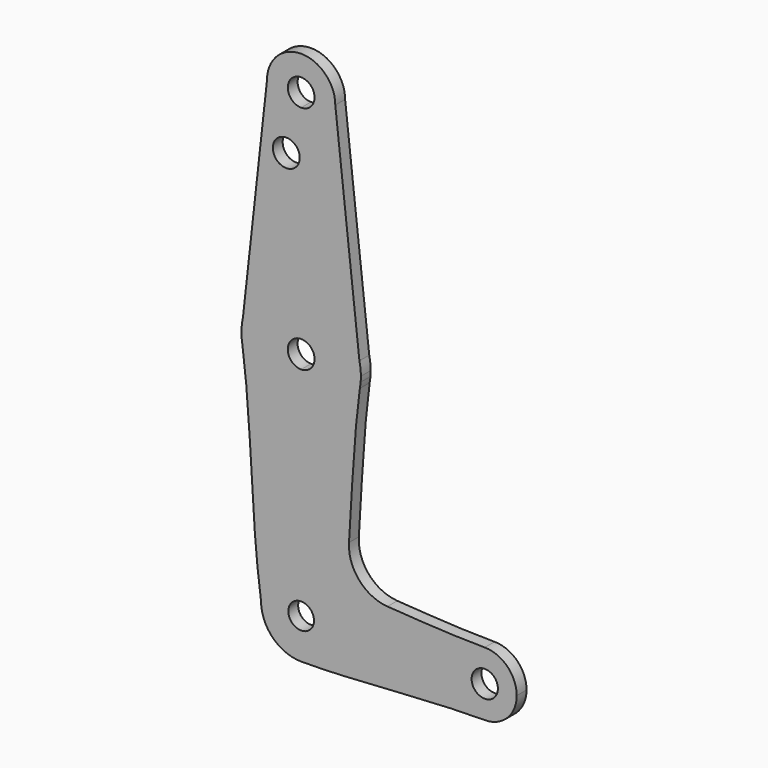
from build123d import *

# Parameters (mm, degrees)
F0_R     = 3.338805446
F1_DEPTH = 3.048


with BuildPart() as f1:
    # F0 (on Front) → F1 (new body)
    with BuildSketch(Plane.XZ):
        with BuildLine():
            ThreePointArc((-48.8398405267, 60.6527402997), (-46.3601680284, 54.6662813241), (-40.3737090528, 52.1866088258))
            ThreePointArc((-40.3737090528, 52.1866088258), (-34.3872500772, 54.6662813241), (-31.9075775789, 60.6527402997))
            ThreePointArc((-31.9075775789, 60.6527402997), (-40.3737090528, 69.1188717736), (-48.8398405267, 60.6527402997))
        make_face()
        with BuildLine():
            ThreePointArc((-37.0553247631, 60.6527402997), (-38.0272570189, 58.3062882658), (-40.3737090528, 57.33435601))
            ThreePointArc((-40.3737090528, 57.33435601), (-42.7201610867, 62.9991923336), (-37.0553247631, 60.6527402997))
        make_face(mode=Mode.SUBTRACT)
        with BuildLine():
            ThreePointArc((-31.9075775789, 60.6527402997), (-34.3872500772, 54.6662813241), (-40.3737090528, 52.1866088258))
            Line((-40.3737090528, 52.1866088258), (-40.3737090528, 18.3121075428))
            ThreePointArc((-40.3737090528, 18.3121075428), (-31.1210192063, 15.0658316355), (-25.9247871381, 6.75019883))
            add(Edge.make_bspline(
                [(-31.9075775789, 60.6527402997), (-29.9133140986, 42.6852264765), (-27.9190506183, 24.7177126532), (-25.9247871381, 6.75019883)],
                knots=[0, 0, 0, 0, 54.2335482737, 54.2335482737, 54.2335482737, 54.2335482737], degree=3))
        make_face()
        with BuildLine():
            Line((-40.3737090528, 18.3121075428), (-40.3737090528, 52.1866088258))
            ThreePointArc((-40.3737090528, 52.1866088258), (-46.3601680284, 54.6662813241), (-48.8398405267, 60.6527402997))
            add(Edge.make_bspline(
                [(-48.8398405267, 60.6527402997), (-50.834104007, 42.6852264765), (-52.8283674873, 24.7177126532), (-54.8226309675, 6.75019883)],
                knots=[0, 0, 0, 0, 54.2335482737, 54.2335482737, 54.2335482737, 54.2335482737], degree=3))
            ThreePointArc((-54.8226309675, 6.75019883), (-49.6263988993, 15.0658316355), (-40.3737090528, 18.3121075428))
        make_face()
        with Locations((-44.0608076751, 46.2730638683)):
            Circle(F0_R, mode=Mode.SUBTRACT)
        with BuildLine():
            ThreePointArc((-25.9247871381, 6.75019883), (-31.1210192063, 15.0658316355), (-40.3737090528, 18.3121075428))
            Line((-40.3737090528, 18.3121075428), (-40.3737090528, 6.825499461))
            ThreePointArc((-40.3737090528, 6.825499461), (-38.0241643353, 5.8522861736), (-37.0509510478, 3.502741456))
            ThreePointArc((-37.0509510478, 3.502741456), (-38.0241643353, 1.1531967385), (-40.3737090528, 0.1799834511))
            Line((-40.3737090528, 0.1799834511), (-40.3737090528, -11.3066246308))
            ThreePointArc((-40.3737090528, -11.3066246308), (-30.9189329127, -7.8957028253), (-25.8194413828, 0.7658423924))
            add(Edge.make_bspline(
                [(-25.6218092077, 2.199370882), (-25.689716363, 1.7216544124), (-25.7555582996, 1.2438093753), (-25.8194413828, 0.7658423924)],
                knots=[0, 0, 0, 0, 1.4434370692, 1.4434370692, 1.4434370692, 1.4434370692], degree=3))
            ThreePointArc((-25.6218092077, 2.199370882), (-25.5787165017, 2.850423048), (-25.564342966, 3.502741456))
            add(Edge.make_bspline(
                [(-25.9247871381, 6.75019883), (-25.8046390807, 5.6677130387), (-25.6844910233, 4.5852272473), (-25.564342966, 3.502741456)],
                knots=[54.2335482737, 54.2335482737, 54.2335482737, 54.2335482737, 57.500947759, 57.500947759, 57.500947759, 57.500947759], degree=3))
        make_face()
        with BuildLine():
            Line((-40.3737090528, 6.825499461), (-40.3737090528, 18.3121075428))
            ThreePointArc((-40.3737090528, 18.3121075428), (-49.6263988993, 15.0658316355), (-54.8226309675, 6.75019883))
            add(Edge.make_bspline(
                [(-54.8226309675, 6.75019883), (-54.9427790249, 5.6677130387), (-55.0629270823, 4.5852272473), (-55.1830751396, 3.502741456)],
                knots=[54.2335482737, 54.2335482737, 54.2335482737, 54.2335482737, 57.500947759, 57.500947759, 57.500947759, 57.500947759], degree=3))
            ThreePointArc((-55.1830751396, 3.502741456), (-55.16469891, 2.7652165843), (-55.1096158257, 2.0295220307))
            add(Edge.make_bspline(
                [(-55.1096158257, 2.0295220307), (-55.0564401475, 1.6554290587), (-55.0045376129, 1.2813360137), (-54.9538568961, 0.9072428986)],
                knots=[0, 0, 0, 0, 1.1264122236, 1.1264122236, 1.1264122236, 1.1264122236], degree=3))
            ThreePointArc((-54.9538568961, 0.9072428986), (-49.8836942152, -7.8496814617), (-40.3737090528, -11.3066246308))
            Line((-40.3737090528, -11.3066246308), (-40.3737090528, 0.1799834511))
            ThreePointArc((-40.3737090528, 0.1799834511), (-43.6964670578, 3.502741456), (-40.3737090528, 6.825499461))
        make_face()
        with BuildLine():
            ThreePointArc((-25.564342966, 3.502741456), (-25.6547298408, 5.1364411987), (-25.9247871381, 6.75019883))
            add(Edge.make_bspline(
                [(-25.9247871381, 6.75019883), (-25.8046390807, 5.6677130387), (-25.6844910233, 4.5852272473), (-25.564342966, 3.502741456)],
                knots=[54.2335482737, 54.2335482737, 54.2335482737, 54.2335482737, 57.500947759, 57.500947759, 57.500947759, 57.500947759], degree=3))
        make_face()
        with BuildLine():
            add(Edge.make_bspline(
                [(-54.8226309675, 6.75019883), (-54.9427790249, 5.6677130387), (-55.0629270823, 4.5852272473), (-55.1830751396, 3.502741456)],
                knots=[54.2335482737, 54.2335482737, 54.2335482737, 54.2335482737, 57.500947759, 57.500947759, 57.500947759, 57.500947759], degree=3))
            ThreePointArc((-54.8226309675, 6.75019883), (-55.0926882648, 5.1364411987), (-55.1830751396, 3.502741456))
        make_face()
        with BuildLine():
            ThreePointArc((-25.8194413828, 0.7658423924), (-30.9189329127, -7.8957028253), (-40.3737090528, -11.3066246308))
            Line((-40.3737090528, -11.3066246308), (-40.3737090528, -43.6920970678))
            add(Edge.make_bspline(
                [(-29.2968091513, -43.9985364744), (-33.0339667691, -43.8142378214), (-36.7371842262, -43.69209709), (-40.3737090528, -43.6920970678)],
                knots=[34.3884430891, 34.3884430891, 34.3884430891, 34.3884430891, 45.5806839994, 45.5806839994, 45.5806839994, 45.5806839994], degree=3))
            add(Edge.make_bspline(
                [(-28.5031349311, -33.745569321), (-28.7247903418, -37.1658958874), (-28.9765210206, -40.5843501576), (-29.2968091568, -43.9985364736)],
                knots=[36.0644801438, 36.0644801438, 36.0644801438, 36.0644801438, 46.3497924724, 46.3497924724, 46.3497924724, 46.3497924724], degree=3))
            add(Edge.make_bspline(
                [(-25.8194413828, 0.7658423924), (-27.3516862062, -10.698263565), (-27.7570281259, -22.2325233774), (-28.5031349311, -33.745569321)],
                knots=[1.4434370692, 1.4434370692, 1.4434370692, 1.4434370692, 36.0644801438, 36.0644801438, 36.0644801438, 36.0644801438], degree=3))
        make_face()
        with BuildLine():
            Line((-40.3737090528, -43.6920970678), (-40.3737090528, -11.3066246308))
            ThreePointArc((-40.3737090528, -11.3066246308), (-49.8836942152, -7.8496814617), (-54.9538568961, 0.9072428986))
            add(Edge.make_bspline(
                [(-54.9538568961, 0.9072428986), (-52.4902517713, -17.2775376799), (-52.9137553274, -35.4624837616), (-50.3288693726, -53.6472573876)],
                knots=[1.1264122236, 1.1264122236, 1.1264122236, 1.1264122236, 55.8816544409, 55.8816544409, 55.8816544409, 55.8816544409], degree=3))
            ThreePointArc((-50.3288693726, -53.6472573876), (-47.4130704227, -46.6078960177), (-40.3737090528, -43.6920970678))
        make_face()
        with BuildLine():
            ThreePointArc((-25.8194413828, 0.7658423924), (-25.703105296, 1.4801912576), (-25.6218092077, 2.199370882))
            add(Edge.make_bspline(
                [(-25.6218092077, 2.199370882), (-25.689716363, 1.7216544124), (-25.7555582996, 1.2438093753), (-25.8194413828, 0.7658423924)],
                knots=[0, 0, 0, 0, 1.4434370692, 1.4434370692, 1.4434370692, 1.4434370692], degree=3))
        make_face()
        with BuildLine():
            add(Edge.make_bspline(
                [(-55.1096158257, 2.0295220307), (-55.0564401475, 1.6554290587), (-55.0045376129, 1.2813360137), (-54.9538568961, 0.9072428986)],
                knots=[0, 0, 0, 0, 1.1264122236, 1.1264122236, 1.1264122236, 1.1264122236], degree=3))
            ThreePointArc((-55.1096158257, 2.0295220307), (-55.0424732194, 1.466892317), (-54.9538568961, 0.9072428986))
        make_face()
        with BuildLine():
            ThreePointArc((-30.418548733, -53.6472573876), (-33.3343476829, -46.6078960177), (-40.3737090528, -43.6920970678))
            Line((-40.3737090528, -43.6920970678), (-40.3737090528, -50.4648009147))
            ThreePointArc((-40.3737090528, -50.4648009147), (-38.1233724999, -51.3969208348), (-37.1912525798, -53.6472573876))
            Line((-37.1912525798, -53.6472573876), (-30.418548733, -53.6472573876))
        make_face()
        with BuildLine():
            add(Edge.make_bspline(
                [(-29.2968091513, -43.9985364744), (-33.0339667691, -43.8142378214), (-36.7371842262, -43.69209709), (-40.3737090528, -43.6920970678)],
                knots=[34.3884430891, 34.3884430891, 34.3884430891, 34.3884430891, 45.5806839994, 45.5806839994, 45.5806839994, 45.5806839994], degree=3))
            ThreePointArc((-40.3737090528, -43.6920970678), (-33.3343476829, -46.6078960177), (-30.418548733, -53.6472573876))
            add(Edge.make_bspline(
                [(-29.2968091568, -43.9985364736), (-29.5989469592, -47.2192450606), (-29.9620922477, -50.4361557069), (-30.418548733, -53.6472573876)],
                knots=[46.3497924724, 46.3497924724, 46.3497924724, 46.3497924724, 56.0522488324, 56.0522488324, 56.0522488324, 56.0522488324], degree=3))
        make_face()
        with BuildLine():
            Line((-40.3737090528, -50.4648009147), (-40.3737090528, -43.6920970678))
            ThreePointArc((-40.3737090528, -43.6920970678), (-47.4130704227, -46.6078960177), (-50.3288693726, -53.6472573876))
            ThreePointArc((-50.3288693726, -53.6472573876), (-47.4130704227, -60.6866187576), (-40.3737090528, -63.6024177074))
            ThreePointArc((-40.3737090528, -63.6024177074), (-33.3343476829, -60.6866187576), (-30.418548733, -53.6472573876))
            Line((-30.418548733, -53.6472573876), (-37.1912525798, -53.6472573876))
            ThreePointArc((-37.1912525798, -53.6472573876), (-42.6240456057, -55.8975939405), (-40.3737090528, -50.4648009147))
        make_face()
        with BuildLine():
            Line((-2.7674630824, -53.6472573876), (-30.418548733, -53.6472573876))
            ThreePointArc((-30.418548733, -53.6472573876), (-33.3343476829, -60.6866187576), (-40.3737090528, -63.6024177074))
            add(Edge.make_bspline(
                [(5.1619368605, -61.5766573305), (-9.6479024117, -61.5766574207), (-25.5638697806, -63.6024176172), (-40.3737090528, -63.6024177074)],
                knots=[0, 0, 0, 0, 45.5806839994, 45.5806839994, 45.5806839994, 45.5806839994], degree=3))
            ThreePointArc((5.1619368605, -61.5766573305), (-0.4449956098, -59.254189858), (-2.7674630824, -53.6472573876))
        make_face()
        with BuildLine():
            add(Edge.make_bspline(
                [(-29.2968091568, -43.9985364736), (-29.5989469592, -47.2192450606), (-29.9620922477, -50.4361557069), (-30.418548733, -53.6472573876)],
                knots=[46.3497924724, 46.3497924724, 46.3497924724, 46.3497924724, 56.0522488324, 56.0522488324, 56.0522488324, 56.0522488324], degree=3))
            Line((-30.418548733, -53.6472573876), (-2.7674630824, -53.6472573876))
            ThreePointArc((-2.7674630824, -53.6472573876), (-0.4449956098, -48.0403249173), (5.1619368605, -45.7178574448))
            add(Edge.make_bspline(
                [(5.1619368605, -45.7178574448), (-2.6797313071, -45.717857397), (-10.8315136759, -45.1499150115), (-18.9650052423, -44.6154703537)],
                knots=[0, 0, 0, 0, 24.1345359803, 24.1345359803, 24.1345359803, 24.1345359803], degree=3))
            add(Edge.make_bspline(
                [(-18.9650052423, -44.6154703537), (-22.4206369172, -44.3884038014), (-25.8729669225, -44.1673839182), (-29.2968091513, -43.9985364744)],
                knots=[24.1345359803, 24.1345359803, 24.1345359803, 24.1345359803, 34.3884430891, 34.3884430891, 34.3884430891, 34.3884430891], degree=3))
        make_face()
        with BuildLine():
            add(Edge.make_bspline(
                [(-28.5031349311, -33.745569321), (-28.7247903418, -37.1658958874), (-28.9765210206, -40.5843501576), (-29.2968091568, -43.9985364736)],
                knots=[36.0644801438, 36.0644801438, 36.0644801438, 36.0644801438, 46.3497924724, 46.3497924724, 46.3497924724, 46.3497924724], degree=3))
            add(Edge.make_bspline(
                [(-18.9650052423, -44.6154703537), (-22.4206369172, -44.3884038014), (-25.8729669225, -44.1673839182), (-29.2968091513, -43.9985364744)],
                knots=[24.1345359803, 24.1345359803, 24.1345359803, 24.1345359803, 34.3884430891, 34.3884430891, 34.3884430891, 34.3884430891], degree=3))
            ThreePointArc((-18.9650052423, -44.6154703537), (-25.9838678208, -41.1546742014), (-28.5031349311, -33.745569321))
        make_face()
        with BuildLine():
            ThreePointArc((5.1619368605, -45.7178574448), (-0.4449956098, -48.0403249173), (-2.7674630824, -53.6472573876))
            ThreePointArc((-2.7674630824, -53.6472573876), (-0.4449956098, -59.254189858), (5.1619368605, -61.5766573305))
            ThreePointArc((5.1619368605, -61.5766573305), (10.7688693309, -59.254189858), (13.0913368034, -53.6472573876))
            ThreePointArc((13.0913368034, -53.6472573876), (10.7688693309, -48.0403249173), (5.1619368605, -45.7178574448))
        make_face()
        with BuildLine():
            ThreePointArc((8.4235029173, -53.6472573876), (5.1619368605, -56.9088234444), (1.9003708038, -53.6472573876))
            ThreePointArc((1.9003708038, -53.6472573876), (5.1619368605, -50.3856913309), (8.4235029173, -53.6472573876))
        make_face(mode=Mode.SUBTRACT)
    extrude(amount=F1_DEPTH)


solid = f1.part
